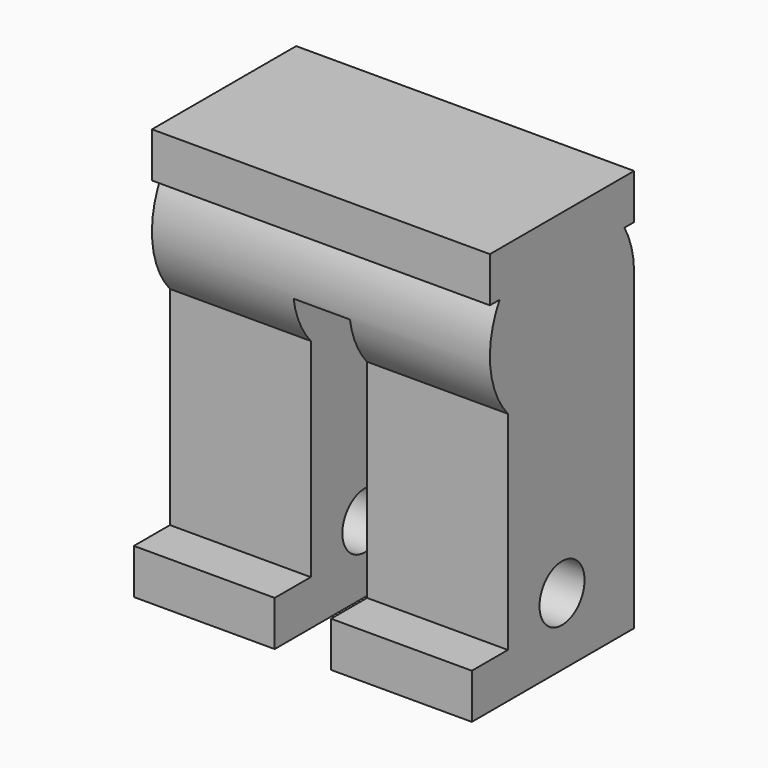
from build123d import *

# Parameters (mm, degrees)
F0_R     = 1.25
F1_DEPTH = 7.5
F2_R     = 11
F3_DEPTH = 1.25


# Not quite as in the source:
# - a feature of the source that left no trace in its solid (it failed there, or was rolled back) is left out


with BuildPart() as f1:
    # F0 (on Right) → F1 (new body, symmetric)
    with BuildSketch(Plane.YZ):
        with BuildLine():
            Line((4, -1), (4, 1))
            Line((4, 1), (-4, 1))
            Line((-4, 1), (-4, -1))
            Line((-4, -1), (-3.4641016151, -1))
            ThreePointArc((-3.4641016151, -1), (-3.9803488917, -3.39600846), (-3.0021324352, -5.6433313908))
            Line((-3.0021324352, -5.6433313908), (-3.0021324352, -14.8694054575))
            Line((-3.0021324352, -14.8694054575), (-5.0021324352, -14.8694054575))
            Line((-5.0021324352, -14.8694054575), (-5.0021324352, -16.8694054575))
            Line((-5.0021324352, -16.8694054575), (3.9978675648, -16.8694054575))
            Line((3.9978675648, -16.8694054575), (3.9978675648, -14.8694054575))
            Line((3.9978675648, -14.8694054575), (3.9978675648, -3.1305945425))
            Line((3.9978675648, -3.1305945425), (3.9978675648, -2.8694054575))
            ThreePointArc((3.9978675648, -2.8694054575), (3.846285897, -1.901781079), (3.4641016151, -1))
            Line((3.4641016151, -1), (4, -1))
        make_face()
        with Locations((0, -13.8694054575)):
            Circle(F0_R, mode=Mode.SUBTRACT)
        with BuildLine():
            ThreePointArc((3.9978675648, -3.1305945425), (4, -3), (3.9978675648, -2.8694054575))
            Line((3.9978675648, -2.8694054575), (3.9978675648, -3.1305945425))
        make_face()
    extrude(amount=F1_DEPTH, both=True)

    # F2 (on Right) → F3 (cut, symmetric)
    with BuildSketch(Plane.YZ):
        with Locations((0, -13.8694054575)):
            Circle(F2_R)
    extrude(amount=F3_DEPTH, both=True, mode=Mode.SUBTRACT)


solid = f1.part
